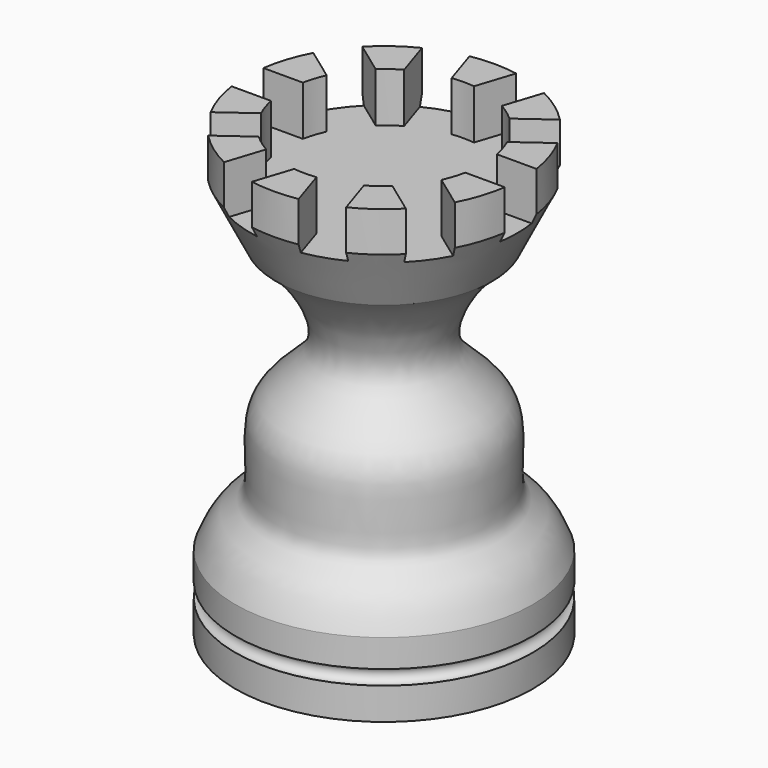
from build123d import *

# Parameters (mm, degrees)
F0_W     = 17.6831819117
F0_H     = 10.16
F2_R     = 12.7
F3_DEPTH = 6.35
F4_W     = 9.8243676867
F4_H     = 5.08
F5_DEPTH = 6.35
F7_R     = 0.9355774764


# Not quite as in the source:
# - a fillet or chamfer that OpenCascade refuses, or shapes differently, is made with other operations: its cross-section is extruded or revolved along the edge and cut away or added


with BuildPart() as f1:
    # F0 (on Front) → F1 (revolve)
    with BuildSketch(Plane.XZ):
        with Locations((8.8415909559, 52.07)):
            Rectangle(F0_W, F0_H)
        with BuildLine():
            Line((0, 46.99), (0, 0))
            Line((0, 0), (19.05, 0))
            Line((19.05, 0), (19.05, 9.525))
            add(Edge.make_bspline(
                [(19.05, 9.525), (17.1376126861, 14.5770803043), (12.2594277566, 14.0530870359), (15.8311377158, 27.1771005404), (4.8442118801, 31.8163009505), (10.984866263, 42.7056935759), (14.4496818428, 44.7679251006), (17.6831819117, 46.99)],
                knots=[0, 0, 0, 0, 0.192461159, 0.3996068615, 0.6001290124, 0.8022738887, 1, 1, 1, 1], degree=3))
            Line((17.6831819117, 46.99), (0, 46.99))
        make_face()
    revolve(axis=Axis((0, 0, 28.575), (0, 0, 1)))

    # F2 (on face) → F3 (cut)
    with BuildSketch(Plane.XY.offset(57.15)):
        Circle(F2_R)
    extrude(amount=-F3_DEPTH, mode=Mode.SUBTRACT)

    # F4 (on face) → F5 (cut)
    with BuildSketch(Plane.XY.offset(57.15)):
        with Locations((15.24, 0)):
            Rectangle(F4_W, F4_H)
        Polygon((6.8624042447, 8.125441191), (9.8483533263, 4.0156348596), (17.7964337439, 9.7902532989), (14.8104846622, 13.9000596303), align=None)
        Polygon((0.7757871558, 10.6072400206), (5.6071542586, 9.0374336892), (8.6430508328, 18.3809625961), (3.81168373, 19.9507689275), align=None)
        Polygon((-5.6071542586, 9.0374336892), (-0.7757871558, 10.6072400206), (-3.81168373, 19.9507689275), (-8.6430508328, 18.3809625961), align=None)
        Polygon((-9.8483533263, 4.0156348596), (-6.8624042447, 8.125441191), (-14.8104846622, 13.9000596303), (-17.7964337439, 9.7902532989), align=None)
        with Locations((-15.24, 0)):
            Rectangle(F4_W, F4_H)
        Polygon((-6.8624042447, -8.125441191), (-9.8483533263, -4.0156348596), (-17.7964337439, -9.7902532989), (-14.8104846622, -13.9000596303), align=None)
        Polygon((-0.7757871558, -10.6072400206), (-5.6071542586, -9.0374336892), (-8.6430508328, -18.3809625961), (-3.81168373, -19.9507689275), align=None)
        Polygon((5.6071542586, -9.0374336892), (0.7757871558, -10.6072400206), (3.81168373, -19.9507689275), (8.6430508328, -18.3809625961), align=None)
        Polygon((9.8483533263, -4.0156348596), (6.8624042447, -8.125441191), (14.8104846622, -13.9000596303), (17.7964337439, -9.7902532989), align=None)
    extrude(amount=-F5_DEPTH, mode=Mode.SUBTRACT)

    # F6: chamfer of 5.08 on 1 edges, made by hand

    # F6_s1 → F6_t2 (revolve, cut)
    with BuildSketch(Plane.XZ):
        with BuildLine():
            Line((13.7794309142, 44.1484930415), (17.7734832624, 52.1998472193))
            Line((17.7734832624, 52.1998472193), (17.8750832624, 52.1998472193))
            ThreePointArc((17.8750832624, 52.1998472193), (17.7847819117, 49.5949236096), (17.7847819117, 46.99))
            Line((17.7847819117, 46.99), (17.7407244212, 46.90626578))
            ThreePointArc((17.7407244212, 46.90626578), (15.7475972656, 45.5454980697), (13.8409013181, 44.0675983603))
            Line((13.8409013181, 44.0675983603), (13.7794309142, 44.1484930415))
        make_face()
    revolve(axis=Axis((0, 0, 46.99), (0, 0, 1)), mode=Mode.SUBTRACT)

    # F7 (on Front) → F8 (revolve, cut)
    with BuildSketch(Plane.XZ):
        with Locations((19.0286766738, 5.0287479535)):
            Circle(F7_R)
    revolve(axis=Axis((0, 0, 5.0287479535), (0, 0, 1)), mode=Mode.SUBTRACT)


solid = f1.part
